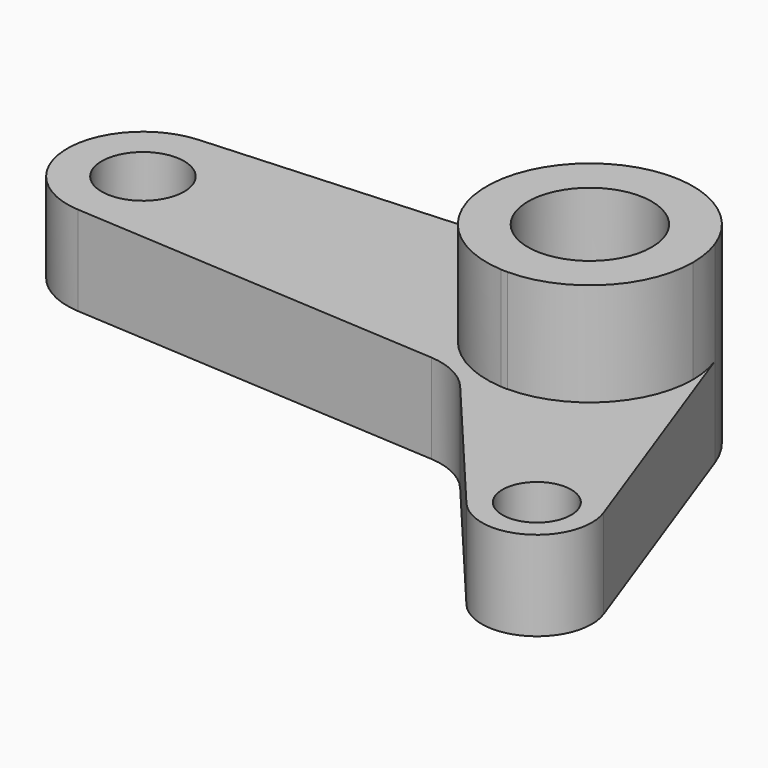
from build123d import *
from build123d import SkipClean  # not in build123d's __all__

# Parameters (mm, degrees)
F0_R     = 5
F0_R_2   = 6
F0_R_3   = 9
F1_DEPTH = 28
F2_R     = 5
F2_R_2   = 6
F3_DEPTH = 10
F4_DEPTH = 25


with BuildPart() as f1:
    # F0 (on Top) → F1 (new body)
    with BuildSketch(Plane.XY):
        with BuildLine():
            ThreePointArc((14.102419126, 5.1109465654), (14.7739007525, 2.5945821542), (15, 0))
            ThreePointArc((15, 0), (10.6066017178, -10.6066017178), (0, -15))
            Line((0, -15), (0, -15.0284832917))
            Line((0, -15.0284832917), (-0.9230769231, -14.9715706923))
            ThreePointArc((-0.9230769231, -14.9715706923), (-15, 3.22e-08), (-0.9230768589, 14.9715706962))
            Line((-0.9230768589, 14.9715706962), (-65.6769230769, 10.979151841))
            ThreePointArc((-65.6769230769, 10.979151841), (-76, 0), (-65.6769230769, -10.979151841))
            Line((-65.6769230769, -10.979151841), (-11.6160346835, -14.3122930019))
            ThreePointArc((-11.6160346835, -14.3122930019), (-7.7343733546, -15.3615666346), (-4.5798065483, -17.8549535065))
            Line((-4.5798065483, -17.8549535065), (13.8787097995, -39.7917254502))
            ThreePointArc((13.8787097995, -39.7917254502), (24, -41.5692193817), (27.5212902005, -31.9151779832))
            Line((27.5212902005, -31.9151779832), (14.102419126, 5.1109465654))
        make_face()
        with Locations((20, -34.6410161514)):
            Circle(F0_R, mode=Mode.SUBTRACT)
        with Locations((-65, 0)):
            Circle(F0_R_2, mode=Mode.SUBTRACT)
        with BuildLine():
            ThreePointArc((0, -15), (10.6066017178, -10.6066017178), (15, 0))
            ThreePointArc((15, 0), (14.7739007525, 2.5945821542), (14.102419126, 5.1109465654))
            ThreePointArc((14.102419126, 5.1109465654), (8.2299296905, 12.5406641486), (-0.9230768589, 14.9715706962))
            ThreePointArc((-0.9230768589, 14.9715706962), (-15, 3.22e-08), (-0.9230769231, -14.9715706923))
            ThreePointArc((-0.9230769231, -14.9715706923), (-0.4617573041, -14.9928909885), (0, -15))
        make_face()
        Circle(F0_R_3, mode=Mode.SUBTRACT)
    extrude(amount=F1_DEPTH)

    # F2 (on face) → F3 (join)
    with BuildSketch(Plane.XY.offset(28)):
        with BuildLine():
            ThreePointArc((14.102419126, 5.1109465654), (14.7739007525, 2.5945821542), (15, 0))
            ThreePointArc((15, 0), (10.6066017178, -10.6066017178), (0, -15))
            Line((0, -15), (0, -15.0284832917))
            Line((0, -15.0284832917), (-0.9230769231, -14.9715706923))
            ThreePointArc((-0.9230769231, -14.9715706923), (-15, 3.22e-08), (-0.9230768589, 14.9715706962))
            Line((-0.9230768589, 14.9715706962), (-65.6769230769, 10.979151841))
            ThreePointArc((-65.6769230769, 10.979151841), (-76, 0), (-65.6769230769, -10.979151841))
            Line((-65.6769230769, -10.979151841), (-11.6160346835, -14.3122930019))
            ThreePointArc((-11.6160346835, -14.3122930019), (-7.7343733546, -15.3615666346), (-4.5798065483, -17.8549535065))
            Line((-4.5798065483, -17.8549535065), (13.8787097995, -39.7917254502))
            ThreePointArc((13.8787097995, -39.7917254502), (24, -41.5692193817), (27.5212902005, -31.9151779832))
            Line((27.5212902005, -31.9151779832), (14.102419126, 5.1109465654))
        make_face()
        with Locations((20, -34.6410161514)):
            Circle(F2_R, mode=Mode.SUBTRACT)
        with Locations((-65, 0)):
            Circle(F2_R_2, mode=Mode.SUBTRACT)
    extrude(amount=F3_DEPTH)

    # F4 (cut): a face of the model
    f4_faces = [f1.faces().sort_by_distance(p)[0] for p in [
        (-23.7772133401, -6.7537112781, 38),
    ]]
    with SkipClean():  # cleaning this boolean's faces spoils the solid; the shape is the same uncleaned
        extrude(f4_faces, amount=-F4_DEPTH, mode=Mode.SUBTRACT)


solid = f1.part
